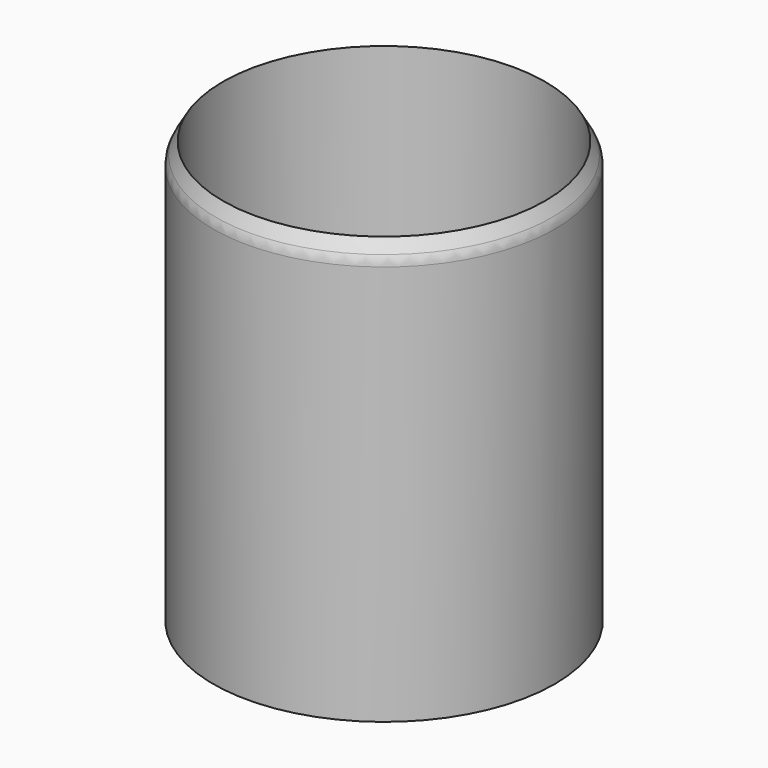
from build123d import *

# Parameters (mm, degrees)
F0_R     = 22.25
F0_R_2   = 21
F1_DEPTH = 55
F2_SIZE2 = 2.165054
F2_SIZE  = 1.24999
F3_R     = 2.5


# Not quite as in the source:
# - a fillet or chamfer is up to 0.001 mm smaller than in the source, because OpenCascade refuses the exact size


with BuildPart() as f1:
    # F0 (on Top) → F1 (new body)
    with BuildSketch(Plane.XY):
        Circle(F0_R)
        Circle(F0_R_2, mode=Mode.SUBTRACT)
    extrude(amount=F1_DEPTH)

    # F2 (size 1.25 and 2.1650635095 in the source; OpenCascade refuses exactly that, so slightly less here)
    f2_edges = [f1.edges().sort_by_distance(p)[0] for p in [
        (-22.25, 0, 55),
    ]]
    f2_side = f1.faces().sort_by_distance((-21.620675, 0, 55))[0]
    chamfer(f2_edges, length=F2_SIZE, length2=F2_SIZE2, reference=f2_side)

    # F3
    f3_edges = [f1.edges().sort_by_distance(p)[0] for p in [
        (-22.25, 0, 52.834946),
    ]]
    fillet(f3_edges, radius=F3_R)


solid = f1.part
